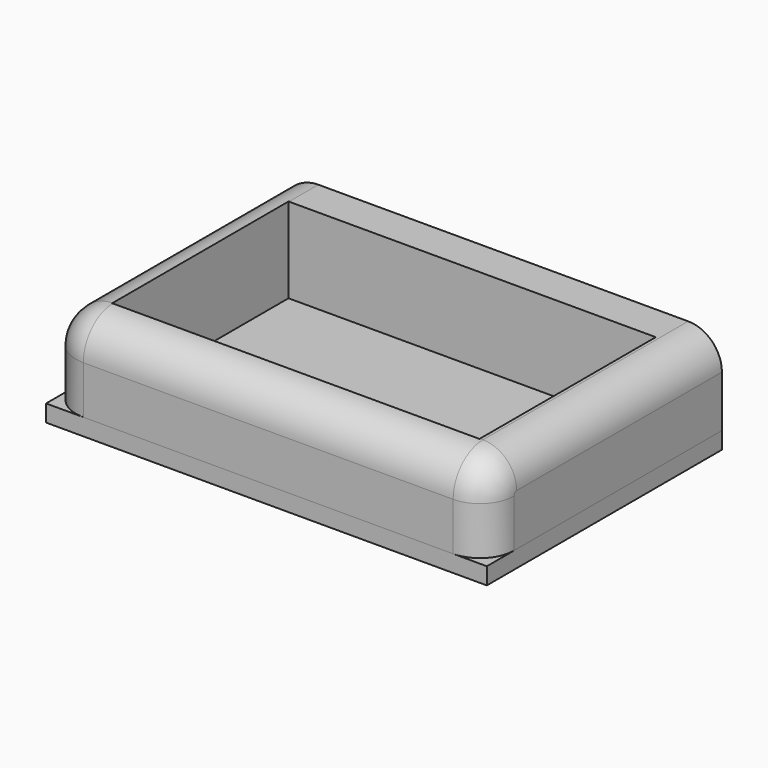
from build123d import *

# Parameters (mm, degrees)
F0_W        = 152.4
F0_H        = 101.6
F0_W_2      = 127
F0_H_2      = 76.2
F1_DEPTH    = 29.464
F2_W        = 152.4
F2_H        = 101.6
F3_DEPTH    = 5.842
F4_T1_DEPTH = 165.9870757085
F5_T1_DEPTH = 171.7161227125
F5_T3_DEPTH = 48.7801227125
F5_T6_ANGLE = 90.0000000015
F6_R        = 11.650994652


# Not quite as in the source:
# - a fillet or chamfer that OpenCascade refuses, or shapes differently, is made with other operations: its cross-section is extruded or revolved along the edge and cut away or added


with BuildPart() as f1:
    # F0 (on Top) → F1 (new body)
    with BuildSketch(Plane.XY):
        Rectangle(F0_W, F0_H)
        Rectangle(F0_W_2, F0_H_2, mode=Mode.SUBTRACT)
    extrude(amount=F1_DEPTH)

    # F4: fillet of radius 12.8774151417 on 1 edges, made by hand

    # F4_s2 → F4_t1 (cut)
    with BuildSketch(Plane.XZ.offset(-82.9935378542)):
        with BuildLine():
            ThreePointArc((-76.2, 16.5865848583), (-72.4282924292, 25.6922924292), (-63.3225848583, 29.464))
            Line((-63.3225848583, 29.464), (-76.2, 29.464))
            Line((-76.2, 29.464), (-76.2, 16.5865848583))
        make_face()
    extrude(amount=F4_T1_DEPTH, mode=Mode.SUBTRACT)

    # F5: fillet of radius 12.8774151417 on 1 edges, made by hand

    # F5_s2 → F5_t1 (cut)
    with BuildSketch(Plane.YZ.offset(-63.3225848583)):
        with BuildLine():
            ThreePointArc((-50.8, 16.5865848583), (-47.0282924292, 25.6922924292), (-37.9225848583, 29.464))
            Line((-37.9225848583, 29.464), (-50.8, 29.464))
            Line((-50.8, 29.464), (-50.8, 16.5865848583))
        make_face()
    extrude(amount=F5_T1_DEPTH, mode=Mode.SUBTRACT)

    # F5_s4 → F5_t3 (cut)
    with BuildSketch(Plane.XY.offset(-32.1935378542)):
        with BuildLine():
            ThreePointArc((-63.3225848583, -50.8), (-72.4282924292, -47.0282924292), (-76.2, -37.9225848583))
            Line((-76.2, -37.9225848583), (-76.2, -50.8))
            Line((-76.2, -50.8), (-63.3225848583, -50.8))
        make_face()
    extrude(amount=F5_T3_DEPTH, mode=Mode.SUBTRACT)

    # F5_s5 → F5_t6 (revolve, cut)
    with BuildSketch(Plane.XY.offset(16.5865848585)):
        with BuildLine():
            ThreePointArc((-63.3225848583, -50.8), (-72.4282924292, -47.0282924292), (-76.2, -37.9225848583))
            Line((-76.2, -37.9225848583), (-76.2, -50.8))
            Line((-76.2, -50.8), (-63.3225848583, -50.8))
        make_face()
    revolve(axis=Axis((-63.3225848585, -50.8, 16.5865848585), (0, 1, 0)), revolution_arc=F5_T6_ANGLE, mode=Mode.SUBTRACT)

    # F6
    f6_edges = [f1.edges().sort_by_distance(p)[0] for p in [
        (76.2, 6.438708, 29.464),
    ]]
    fillet(f6_edges, radius=F6_R)


with BuildPart() as f3:
    # F2 (on Top) → F3 (new body)
    with BuildSketch(Plane.XY):
        Rectangle(F2_W, F2_H)
    extrude(amount=-F3_DEPTH)


solid = Compound([f1.part, f3.part])
